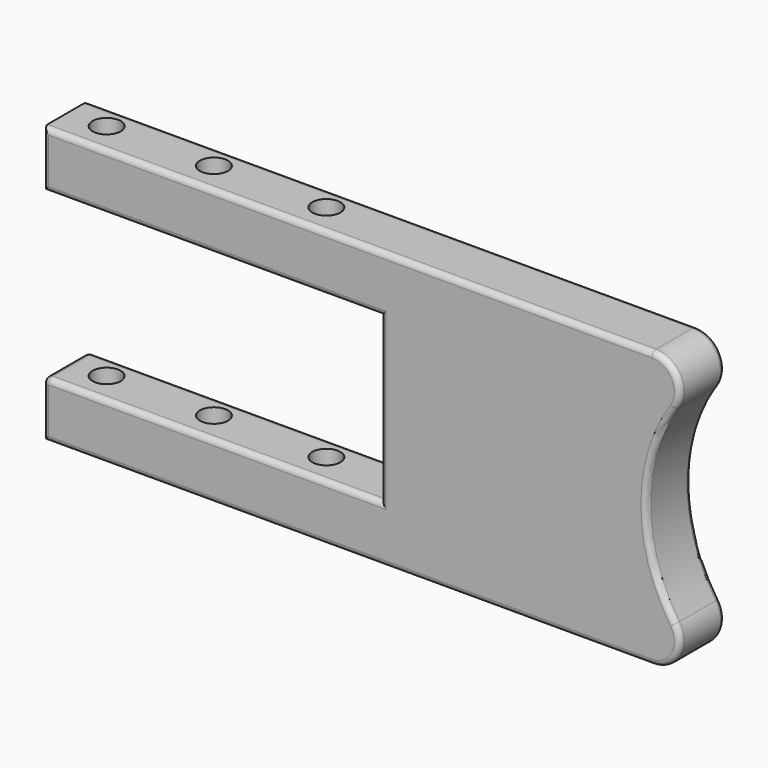
from build123d import *

# Parameters (mm, degrees)
F1_DEPTH     = 12.7
F2_R         = 6.35
F3_W         = 76.2
F3_H         = 36.9506594684
F4_DEPTH     = 12.701
F5_R         = 3.175
F6_DEPTH     = 62.3516594684
F7_T1_DEPTH  = 140.6081975657
F7_T3_DEPTH  = 79.3774143709
F7_T5_DEPTH  = 36.9506594684
F7_T7_DEPTH  = 74.9290343146
F7_T9_DEPTH  = 19.0548287418
F7_T11_DEPTH = 14.6064486855
F7_T13_DEPTH = 10.1580686292
F7_S17_W     = 1.3985022539
F7_S17_H     = 1.3985022539
F7_T18_DEPTH = 1.398502254
F7_S23_W     = 1.3985022539
F7_S23_H     = 1.3985022539
F7_T24_DEPTH = 1.398502254
F7_T40_ANGLE = 123.952133453
F7_T42_ANGLE = 67.904266906
F7_T44_ANGLE = 123.952133453
F7_T46_ANGLE = 123.952133453
F7_T48_ANGLE = 67.904266906
F7_T50_ANGLE = 123.952133453
F7_T55_DEPTH = 40.1280738393
F7_T59_DEPTH = 82.5548287418
F7_T66_DEPTH = 78.1064486855
F7_T70_DEPTH = 40.1280738393
F7_T77_DEPTH = 78.1064486855
F7_T81_DEPTH = 40.1280738393
F7_T88_DEPTH = 40.1280738393
F7_T92_DEPTH = 82.5548287418


# Not quite as in the source:
# - a fillet or chamfer that OpenCascade refuses, or shapes differently, is made with other operations: its cross-section is extruded or revolved along the edge and cut away or added


with BuildPart() as f1:
    # F0 (on Front) → F1 (new body)
    with BuildSketch(Plane.XZ):
        with BuildLine():
            Line((152.4, 62.3506594684), (0, 62.3506594684))
            Line((0, 62.3506594684), (0, 0))
            Line((0, 0), (152.4, 0))
            ThreePointArc((152.4, 0), (136.2022559561, 31.1753297342), (152.4, 62.3506594684))
        make_face()
    extrude(amount=F1_DEPTH)

    # F2
    f2_edges = [f1.edges().sort_by_distance(p)[0] for p in [
        (152.4, -6.35, 62.350659),
        (152.4, -6.35, 0),
    ]]
    fillet(f2_edges, radius=F2_R)

    # F3 (on face) → F4 (cut, through all)
    with BuildSketch(Plane.XZ.offset(12.7)):
        with Locations((38.1, 31.1753297342)):
            Rectangle(F3_W, F3_H)
    extrude(amount=-F4_DEPTH, mode=Mode.SUBTRACT)

    # F5 (on face) → F6 (cut, through all)
    with BuildSketch(Plane(origin=(0, 0, 0), x_dir=(1, 0, 0), z_dir=(0, 0, -1))):
        with Locations((58.1839601433, 5.4876524955)):
            Circle(F5_R)
        with Locations((32.7839601433, 5.4876524955)):
            Circle(F5_R)
        with Locations((8.5653553438, 5.4876524955)):
            Circle(F5_R)
    extrude(amount=-F6_DEPTH, mode=Mode.SUBTRACT)

    # F7: fillet of radius 1.27 on 19 edges, made by hand

    # F7_s2 → F7_t1 (cut)
    with BuildSketch(Plane.YZ.offset(-3.1774143709)):
        with BuildLine():
            ThreePointArc((-12.7004, 61.079693783), (-12.3280256121, 61.9786850805), (-11.4290343146, 62.3510594684))
            Line((-11.4290343146, 62.3510594684), (-11.4290343146, 62.4781960369))
            ThreePointArc((-11.4290343146, 62.4781960369), (-12.0645171573, 62.4777960369), (-12.7, 62.4777960369))
            Line((-12.7, 62.4777960369), (-12.8271365685, 62.3506594684))
            ThreePointArc((-12.8271365685, 62.3506594684), (-12.8271365685, 61.7151766257), (-12.8275365685, 61.079693783))
            Line((-12.8275365685, 61.079693783), (-12.7004, 61.079693783))
        make_face()
        with BuildLine():
            ThreePointArc((0.0004, 1.2709656854), (-0.3719743879, 0.3719743879), (-1.2709656854, -0.0004))
            Line((-1.2709656854, -0.0004), (-1.2709656854, -0.1275365685))
            ThreePointArc((-1.2709656854, -0.1275365685), (-0.6354828427, -0.1271365685), (0, -0.1271365685))
            Line((0, -0.1271365685), (0.1271365685, 0))
            ThreePointArc((0.1271365685, 0), (0.1271365685, 0.6354828427), (0.1275365685, 1.2709656854))
            Line((0.1275365685, 1.2709656854), (0.0004, 1.2709656854))
        make_face()
        with BuildLine():
            ThreePointArc((0.0004, 61.079693783), (-0.3719743879, 61.9786850805), (-1.2709656854, 62.3510594684))
            Line((-1.2709656854, 62.3510594684), (-1.2709656854, 62.4781960369))
            ThreePointArc((-1.2709656854, 62.4781960369), (-0.6354828427, 62.4777960369), (0, 62.4777960369))
            Line((0, 62.4777960369), (0.1271365685, 62.3506594684))
            ThreePointArc((0.1271365685, 62.3506594684), (0.1271365685, 61.7151766257), (0.1275365685, 61.079693783))
            Line((0.1275365685, 61.079693783), (0.0004, 61.079693783))
        make_face()
        with BuildLine():
            ThreePointArc((-12.7004, 1.2709656854), (-12.3280256121, 0.3719743879), (-11.4290343146, -0.0004))
            Line((-11.4290343146, -0.0004), (-11.4290343146, -0.1275365685))
            ThreePointArc((-11.4290343146, -0.1275365685), (-12.0645171573, -0.1271365685), (-12.7, -0.1271365685))
            Line((-12.7, -0.1271365685), (-12.8271365685, 0))
            ThreePointArc((-12.8271365685, 0), (-12.8271365685, 0.6354828427), (-12.8275365685, 1.2709656854))
            Line((-12.8275365685, 1.2709656854), (-12.7004, 1.2709656854))
        make_face()
    extrude(amount=F7_T1_DEPTH, mode=Mode.SUBTRACT)

    # F7_s4 → F7_t3 (cut)
    with BuildSketch(Plane.YZ.offset(-3.1774143709)):
        with BuildLine():
            ThreePointArc((-12.7004, 50.9216251538), (-12.3280256121, 50.0226338563), (-11.4290343146, 49.6502594684))
            Line((-11.4290343146, 49.6502594684), (-11.4290343146, 49.5231228998))
            ThreePointArc((-11.4290343146, 49.5231228998), (-12.0645171573, 49.5235228998), (-12.7, 49.5235228998))
            Line((-12.7, 49.5235228998), (-12.8271365685, 49.6506594684))
            ThreePointArc((-12.8271365685, 49.6506594684), (-12.8271365685, 50.2861423111), (-12.8275365685, 50.9216251538))
            Line((-12.8275365685, 50.9216251538), (-12.7004, 50.9216251538))
        make_face()
        with BuildLine():
            ThreePointArc((0.0004, 50.9216251538), (-0.3719743879, 50.0226338563), (-1.2709656854, 49.6502594684))
            Line((-1.2709656854, 49.6502594684), (-1.2709656854, 49.5231228998))
            ThreePointArc((-1.2709656854, 49.5231228998), (-0.6354828427, 49.5235228998), (0, 49.5235228998))
            Line((0, 49.5235228998), (0.1271365685, 49.6506594684))
            ThreePointArc((0.1271365685, 49.6506594684), (0.1271365685, 50.2861423111), (0.1275365685, 50.9216251538))
            Line((0.1275365685, 50.9216251538), (0.0004, 50.9216251538))
        make_face()
    extrude(amount=F7_T3_DEPTH, mode=Mode.SUBTRACT)

    # F7_s6 → F7_t5 (cut)
    with BuildSketch(Plane.XY.offset(12.7)):
        with BuildLine():
            ThreePointArc((77.4709656854, -12.7004), (76.5719743879, -12.3280256121), (76.1996, -11.4290343146))
            Line((76.1996, -11.4290343146), (76.0724634315, -11.4290343146))
            ThreePointArc((76.0724634315, -11.4290343146), (76.0728634315, -12.0645171573), (76.0728634315, -12.7))
            Line((76.0728634315, -12.7), (76.2, -12.8271365685))
            ThreePointArc((76.2, -12.8271365685), (76.8354828427, -12.8271365685), (77.4709656854, -12.8275365685))
            Line((77.4709656854, -12.8275365685), (77.4709656854, -12.7004))
        make_face()
        with BuildLine():
            ThreePointArc((77.4709656854, 0.0004), (76.5719743879, -0.3719743879), (76.1996, -1.2709656854))
            Line((76.1996, -1.2709656854), (76.0724634315, -1.2709656854))
            ThreePointArc((76.0724634315, -1.2709656854), (76.0728634315, -0.6354828427), (76.0728634315, 0))
            Line((76.0728634315, 0), (76.2, 0.1271365685))
            ThreePointArc((76.2, 0.1271365685), (76.8354828427, 0.1271365685), (77.4709656854, 0.1275365685))
            Line((77.4709656854, 0.1275365685), (77.4709656854, 0.0004))
        make_face()
    extrude(amount=F7_T5_DEPTH, mode=Mode.SUBTRACT)

    # F7_s8 → F7_t7 (cut)
    with BuildSketch(Plane.YZ.offset(1.2709656854)):
        with BuildLine():
            ThreePointArc((-12.7004, 11.4290343146), (-12.3280256121, 12.3280256121), (-11.4290343146, 12.7004))
            Line((-11.4290343146, 12.7004), (-11.4290343146, 12.8275365685))
            ThreePointArc((-11.4290343146, 12.8275365685), (-12.0645171573, 12.8271365685), (-12.7, 12.8271365685))
            Line((-12.7, 12.8271365685), (-12.8271365685, 12.7))
            ThreePointArc((-12.8271365685, 12.7), (-12.8271365685, 12.0645171573), (-12.8275365685, 11.4290343146))
            Line((-12.8275365685, 11.4290343146), (-12.7004, 11.4290343146))
        make_face()
        with BuildLine():
            ThreePointArc((0.0004, 11.4290343146), (-0.3719743879, 12.3280256121), (-1.2709656854, 12.7004))
            Line((-1.2709656854, 12.7004), (-1.2709656854, 12.8275365685))
            ThreePointArc((-1.2709656854, 12.8275365685), (-0.6354828427, 12.8271365685), (0, 12.8271365685))
            Line((0, 12.8271365685), (0.1271365685, 12.7))
            ThreePointArc((0.1271365685, 12.7), (0.1271365685, 12.0645171573), (0.1275365685, 11.4290343146))
            Line((0.1275365685, 11.4290343146), (0.0004, 11.4290343146))
        make_face()
    extrude(amount=F7_T7_DEPTH, mode=Mode.SUBTRACT)

    # F7_s10 → F7_t9 (cut)
    with BuildSketch(Plane.XY.offset(46.4732450975)):
        with BuildLine():
            ThreePointArc((1.2709656854, -12.7004), (0.3719743879, -12.3280256121), (-0.0004, -11.4290343146))
            Line((-0.0004, -11.4290343146), (-0.1275365685, -11.4290343146))
            ThreePointArc((-0.1275365685, -11.4290343146), (-0.1271365685, -12.0645171573), (-0.1271365685, -12.7))
            Line((-0.1271365685, -12.7), (0, -12.8271365685))
            ThreePointArc((0, -12.8271365685), (0.6354828427, -12.8271365685), (1.2709656854, -12.8275365685))
            Line((1.2709656854, -12.8275365685), (1.2709656854, -12.7004))
        make_face()
        with BuildLine():
            ThreePointArc((1.2709656854, 0.0004), (0.3719743879, -0.3719743879), (-0.0004, -1.2709656854))
            Line((-0.0004, -1.2709656854), (-0.1275365685, -1.2709656854))
            ThreePointArc((-0.1275365685, -1.2709656854), (-0.1271365685, -0.6354828427), (-0.1271365685, 0))
            Line((-0.1271365685, 0), (0, 0.1271365685))
            ThreePointArc((0, 0.1271365685), (0.6354828427, 0.1271365685), (1.2709656854, 0.1275365685))
            Line((1.2709656854, 0.1275365685), (1.2709656854, 0.0004))
        make_face()
    extrude(amount=F7_T9_DEPTH, mode=Mode.SUBTRACT)

    # F7_s12 → F7_t11 (cut)
    with BuildSketch(Plane.XY.offset(-3.1774143709)):
        with BuildLine():
            ThreePointArc((1.2709656854, -12.7004), (0.3719743879, -12.3280256121), (-0.0004, -11.4290343146))
            Line((-0.0004, -11.4290343146), (-0.1275365685, -11.4290343146))
            ThreePointArc((-0.1275365685, -11.4290343146), (-0.1271365685, -12.0645171573), (-0.1271365685, -12.7))
            Line((-0.1271365685, -12.7), (0, -12.8271365685))
            ThreePointArc((0, -12.8271365685), (0.6354828427, -12.8271365685), (1.2709656854, -12.8275365685))
            Line((1.2709656854, -12.8275365685), (1.2709656854, -12.7004))
        make_face()
        with BuildLine():
            ThreePointArc((1.2709656854, 0.0004), (0.3719743879, -0.3719743879), (-0.0004, -1.2709656854))
            Line((-0.0004, -1.2709656854), (-0.1275365685, -1.2709656854))
            ThreePointArc((-0.1275365685, -1.2709656854), (-0.1271365685, -0.6354828427), (-0.1271365685, 0))
            Line((-0.1271365685, 0), (0, 0.1271365685))
            ThreePointArc((0, 0.1271365685), (0.6354828427, 0.1271365685), (1.2709656854, 0.1275365685))
            Line((1.2709656854, 0.1275365685), (1.2709656854, 0.0004))
        make_face()
    extrude(amount=F7_T11_DEPTH, mode=Mode.SUBTRACT)

    # F7_s14 → F7_t13 (cut)
    with BuildSketch(Plane.XZ.offset(1.2709656854)):
        with BuildLine():
            ThreePointArc((-0.0004, 11.4290343146), (0.3719743879, 12.3280256121), (1.2709656854, 12.7004))
            Line((1.2709656854, 12.7004), (1.2709656854, 12.8275365685))
            ThreePointArc((1.2709656854, 12.8275365685), (0.6354828427, 12.8271365685), (0, 12.8271365685))
            Line((0, 12.8271365685), (-0.1271365685, 12.7))
            ThreePointArc((-0.1271365685, 12.7), (-0.1271365685, 12.0645171573), (-0.1275365685, 11.4290343146))
            Line((-0.1275365685, 11.4290343146), (-0.0004, 11.4290343146))
        make_face()
    extrude(amount=F7_T13_DEPTH, mode=Mode.SUBTRACT)


with BuildPart() as f7_tool16:
    # F7_s17 → F7_t18 (new body)
    with BuildSketch(Plane.XZ.offset(11.4290343146)):
        with Locations((0.5717145584, 12.1282854416)):
            Rectangle(F7_S17_W, F7_S17_H)
    extrude(amount=F7_T18_DEPTH)

    # F7_s19 → F7_t20 (revolve, cut)
    with BuildSketch(Plane(origin=(1.2709656854, -11.4290343146, 11.4290343146), x_dir=(0.7071067812, 0, -0.7071067812), z_dir=(-0.7071067812, 0, -0.7071067812))):
        with BuildLine():
            ThreePointArc((0, -1.2713656854), (1.2713656854, 0), (0, 1.2713656854))
            Line((0, 1.2713656854), (0, -1.2713656854))
        make_face()
    revolve(axis=Axis((1.2709656854, -11.4290343146, 11.4290343146), (0, -1, 0)), mode=Mode.SUBTRACT)


with BuildPart() as f1_1:
    add(f1.part)

    # F7_t15: cut F7_tool16
    add(f7_tool16.part, mode=Mode.SUBTRACT)


with BuildPart() as f7_tool22:
    # F7_s23 → F7_t24 (new body)
    with BuildSketch(Plane.XZ.offset(1.2709656854)):
        with Locations((0.5717145584, 12.1282854416)):
            Rectangle(F7_S23_W, F7_S23_H)
    extrude(amount=-F7_T24_DEPTH)

    # F7_s25 → F7_t26 (revolve, cut)
    with BuildSketch(Plane(origin=(1.2709656854, -1.2709656854, 11.4290343146), x_dir=(0.7071067812, 0, -0.7071067812), z_dir=(0.7071067812, 0, 0.7071067812))):
        with BuildLine():
            ThreePointArc((0, -1.2713656854), (1.2713656854, 0), (0, 1.2713656854))
            Line((0, 1.2713656854), (0, -1.2713656854))
        make_face()
    revolve(axis=Axis((1.2709656854, -1.2709656854, 11.4290343146), (0, 1, 0)), mode=Mode.SUBTRACT)


with BuildPart() as f1_2:
    add(f1_1.part)

    # F7_t21: cut F7_tool22
    add(f7_tool22.part, mode=Mode.SUBTRACT)

    # F7_s27 → F7_t28 (revolve, cut)
    with BuildSketch(Plane.XZ.offset(5.4876524955)):
        with BuildLine():
            ThreePointArc((62.6299258287, -0.0004), (61.7309345312, 0.3719743879), (61.3585601433, 1.2709656854))
            Line((61.3585601433, 1.2709656854), (61.2314235747, 1.2709656854))
            ThreePointArc((61.2314235747, 1.2709656854), (61.2318235747, 0.6354828427), (61.2318235747, 0))
            Line((61.2318235747, 0), (61.3589601433, -0.1271365685))
            ThreePointArc((61.3589601433, -0.1271365685), (61.994442986, -0.1271365685), (62.6299258287, -0.1275365685))
            Line((62.6299258287, -0.1275365685), (62.6299258287, -0.0004))
        make_face()
    revolve(axis=Axis((58.1839601433, -5.4876524955, 0), (0, 0, -1)), mode=Mode.SUBTRACT)

    # F7_s29 → F7_t30 (revolve, cut)
    with BuildSketch(Plane.XZ.offset(5.4876524955)):
        with BuildLine():
            ThreePointArc((37.2299258287, -0.0004), (36.3309345312, 0.3719743879), (35.9585601433, 1.2709656854))
            Line((35.9585601433, 1.2709656854), (35.8314235747, 1.2709656854))
            ThreePointArc((35.8314235747, 1.2709656854), (35.8318235747, 0.6354828427), (35.8318235747, 0))
            Line((35.8318235747, 0), (35.9589601433, -0.1271365685))
            ThreePointArc((35.9589601433, -0.1271365685), (36.594442986, -0.1271365685), (37.2299258287, -0.1275365685))
            Line((37.2299258287, -0.1275365685), (37.2299258287, -0.0004))
        make_face()
    revolve(axis=Axis((32.7839601433, -5.4876524955, 0), (0, 0, -1)), mode=Mode.SUBTRACT)

    # F7_s31 → F7_t32 (revolve, cut)
    with BuildSketch(Plane.XZ.offset(5.4876524955)):
        with BuildLine():
            ThreePointArc((13.0113210292, -0.0004), (12.1123297316, 0.3719743879), (11.7399553438, 1.2709656854))
            Line((11.7399553438, 1.2709656854), (11.6128187752, 1.2709656854))
            ThreePointArc((11.6128187752, 1.2709656854), (11.6132187752, 0.6354828427), (11.6132187752, 0))
            Line((11.6132187752, 0), (11.7403553438, -0.1271365685))
            ThreePointArc((11.7403553438, -0.1271365685), (12.3758381865, -0.1271365685), (13.0113210292, -0.1275365685))
            Line((13.0113210292, -0.1275365685), (13.0113210292, -0.0004))
        make_face()
    revolve(axis=Axis((8.5653553438, -5.4876524955, 0), (0, 0, -1)), mode=Mode.SUBTRACT)

    # F7_s33 → F7_t34 (revolve, cut)
    with BuildSketch(Plane.XZ.offset(5.4876524955)):
        with BuildLine():
            ThreePointArc((62.6299258287, 49.6502594684), (61.7309345312, 50.0226338563), (61.3585601433, 50.9216251538))
            Line((61.3585601433, 50.9216251538), (61.2314235747, 50.9216251538))
            ThreePointArc((61.2314235747, 50.9216251538), (61.2318235747, 50.2861423111), (61.2318235747, 49.6506594684))
            Line((61.2318235747, 49.6506594684), (61.3589601433, 49.5235228998))
            ThreePointArc((61.3589601433, 49.5235228998), (61.994442986, 49.5235228998), (62.6299258287, 49.5231228998))
            Line((62.6299258287, 49.5231228998), (62.6299258287, 49.6502594684))
        make_face()
    revolve(axis=Axis((58.1839601433, -5.4876524955, 49.6506594684), (0, 0, -1)), mode=Mode.SUBTRACT)

    # F7_s35 → F7_t36 (revolve, cut)
    with BuildSketch(Plane.XZ.offset(5.4876524955)):
        with BuildLine():
            ThreePointArc((37.2299258287, 49.6502594684), (36.3309345312, 50.0226338563), (35.9585601433, 50.9216251538))
            Line((35.9585601433, 50.9216251538), (35.8314235747, 50.9216251538))
            ThreePointArc((35.8314235747, 50.9216251538), (35.8318235747, 50.2861423111), (35.8318235747, 49.6506594684))
            Line((35.8318235747, 49.6506594684), (35.9589601433, 49.5235228998))
            ThreePointArc((35.9589601433, 49.5235228998), (36.594442986, 49.5235228998), (37.2299258287, 49.5231228998))
            Line((37.2299258287, 49.5231228998), (37.2299258287, 49.6502594684))
        make_face()
    revolve(axis=Axis((32.7839601433, -5.4876524955, 49.6506594684), (0, 0, -1)), mode=Mode.SUBTRACT)

    # F7_s37 → F7_t38 (revolve, cut)
    with BuildSketch(Plane.XZ.offset(5.4876524955)):
        with BuildLine():
            ThreePointArc((13.0113210292, 49.6502594684), (12.1123297316, 50.0226338563), (11.7399553438, 50.9216251538))
            Line((11.7399553438, 50.9216251538), (11.6128187752, 50.9216251538))
            ThreePointArc((11.6128187752, 50.9216251538), (11.6132187752, 50.2861423111), (11.6132187752, 49.6506594684))
            Line((11.6132187752, 49.6506594684), (11.7403553438, 49.5235228998))
            ThreePointArc((11.7403553438, 49.5235228998), (12.3758381865, 49.5235228998), (13.0113210292, 49.5231228998))
            Line((13.0113210292, 49.5231228998), (13.0113210292, 49.6502594684))
        make_face()
    revolve(axis=Axis((8.5653553438, -5.4876524955, 49.6506594684), (0, 0, -1)), mode=Mode.SUBTRACT)

    # F7_s39 → F7_t40 (revolve, cut)
    with BuildSketch(Plane(origin=(39.9259181111, 0, -59.2994098312), x_dir=(0, 1, 0), z_dir=(-0.5585001065, 0, 0.8295044491))):
        with BuildLine():
            ThreePointArc((0.0004, -122.6249560906), (-0.3719743879, -123.5239473881), (-1.2709656854, -123.896321776))
            Line((-1.2709656854, -123.896321776), (-1.2709656854, -124.0234583445))
            ThreePointArc((-1.2709656854, -124.0234583445), (-0.6354828427, -124.0230583445), (0, -124.0230583445))
            Line((0, -124.0230583445), (0.1271365685, -123.895921776))
            ThreePointArc((0.1271365685, -123.895921776), (0.1271365685, -123.2604389333), (0.1275365685, -122.6249560906))
            Line((0.1275365685, -122.6249560906), (0.0004, -122.6249560906))
        make_face()
    revolve(axis=Axis((137.4307831947, 0, 6.35), (0, 1, 0)), revolution_arc=F7_T40_ANGLE, mode=Mode.SUBTRACT)

    # F7_s41 → F7_t42 (revolve, cut)
    with BuildSketch(Plane(origin=(39.9259181111, 0, -59.2994098312), x_dir=(0, 1, 0), z_dir=(0.5585001065, 0, -0.8295044491))):
        with BuildLine():
            ThreePointArc((-1.2709656854, 123.896321776), (-0.3719743879, 123.5239473881), (0.0004, 122.6249560906))
            Line((0.0004, 122.6249560906), (0.1275365685, 122.6249560906))
            ThreePointArc((0.1275365685, 122.6249560906), (0.1271365685, 123.2604389333), (0.1271365685, 123.895921776))
            Line((0.1271365685, 123.895921776), (0, 124.0230583445))
            ThreePointArc((0, 124.0230583445), (-0.6354828427, 124.0230583445), (-1.2709656854, 124.0234583445))
            Line((-1.2709656854, 124.0234583445), (-1.2709656854, 123.896321776))
        make_face()
    revolve(axis=Axis((174.3022559561, 0, 31.1753297342), (0, 1, 0)), revolution_arc=F7_T42_ANGLE, mode=Mode.SUBTRACT)

    # F7_s43 → F7_t44 (revolve, cut)
    with BuildSketch(Plane(origin=(68.8116270772, 0, 102.2015038916), x_dir=(0, 1, 0), z_dir=(-0.5585001065, 0, -0.8295044491))):
        with BuildLine():
            ThreePointArc((0.0004, 87.8021061368), (-0.3719743879, 88.7010974343), (-1.2709656854, 89.0734718222))
            Line((-1.2709656854, 89.0734718222), (-1.2709656854, 89.2006083907))
            ThreePointArc((-1.2709656854, 89.2006083907), (-0.6354828427, 89.2002083907), (0, 89.2002083907))
            Line((0, 89.2002083907), (0.1271365685, 89.0730718222))
            ThreePointArc((0.1271365685, 89.0730718222), (0.1271365685, 88.4375889795), (0.1275365685, 87.8021061368))
            Line((0.1275365685, 87.8021061368), (0.0004, 87.8021061368))
        make_face()
    revolve(axis=Axis((137.4307831947, 0, 56.0006594684), (0, -1, 0)), revolution_arc=F7_T44_ANGLE, mode=Mode.SUBTRACT)

    # F7_s45 → F7_t46 (revolve, cut)
    with BuildSketch(Plane(origin=(68.8116270772, 0, 102.2015038916), x_dir=(0, 1, 0), z_dir=(-0.5585001065, 0, -0.8295044491))):
        with BuildLine():
            ThreePointArc((-11.4290343146, 89.0734718222), (-12.3280256121, 88.7010974343), (-12.7004, 87.8021061368))
            Line((-12.7004, 87.8021061368), (-12.8275365685, 87.8021061368))
            ThreePointArc((-12.8275365685, 87.8021061368), (-12.8271365685, 88.4375889795), (-12.8271365685, 89.0730718222))
            Line((-12.8271365685, 89.0730718222), (-12.7, 89.2002083907))
            ThreePointArc((-12.7, 89.2002083907), (-12.0645171573, 89.2002083907), (-11.4290343146, 89.2006083907))
            Line((-11.4290343146, 89.2006083907), (-11.4290343146, 89.0734718222))
        make_face()
    revolve(axis=Axis((137.4307831947, -12.7, 56.0006594684), (0, -1, 0)), revolution_arc=F7_T46_ANGLE, mode=Mode.SUBTRACT)

    # F7_s47 → F7_t48 (revolve, cut)
    with BuildSketch(Plane(origin=(39.9259181111, 0, -59.2994098312), x_dir=(0, 1, 0), z_dir=(0.5585001065, 0, -0.8295044491))):
        with BuildLine():
            ThreePointArc((-11.4290343146, 123.896321776), (-12.3280256121, 123.5239473881), (-12.7004, 122.6249560906))
            Line((-12.7004, 122.6249560906), (-12.8275365685, 122.6249560906))
            ThreePointArc((-12.8275365685, 122.6249560906), (-12.8271365685, 123.2604389333), (-12.8271365685, 123.895921776))
            Line((-12.8271365685, 123.895921776), (-12.7, 124.0230583445))
            ThreePointArc((-12.7, 124.0230583445), (-12.0645171573, 124.0230583445), (-11.4290343146, 124.0234583445))
            Line((-11.4290343146, 124.0234583445), (-11.4290343146, 123.896321776))
        make_face()
    revolve(axis=Axis((174.3022559561, -12.7, 31.1753297342), (0, 1, 0)), revolution_arc=F7_T48_ANGLE, mode=Mode.SUBTRACT)

    # F7_s49 → F7_t50 (revolve, cut)
    with BuildSketch(Plane(origin=(39.9259181111, 0, -59.2994098312), x_dir=(0, 1, 0), z_dir=(-0.5585001065, 0, 0.8295044491))):
        with BuildLine():
            ThreePointArc((-11.4290343146, -123.896321776), (-12.3280256121, -123.5239473881), (-12.7004, -122.6249560906))
            Line((-12.7004, -122.6249560906), (-12.8275365685, -122.6249560906))
            ThreePointArc((-12.8275365685, -122.6249560906), (-12.8271365685, -123.2604389333), (-12.8271365685, -123.895921776))
            Line((-12.8271365685, -123.895921776), (-12.7, -124.0230583445))
            ThreePointArc((-12.7, -124.0230583445), (-12.0645171573, -124.0230583445), (-11.4290343146, -124.0234583445))
            Line((-11.4290343146, -124.0234583445), (-11.4290343146, -123.896321776))
        make_face()
    revolve(axis=Axis((137.4307831947, -12.7, 6.35), (0, 1, 0)), revolution_arc=F7_T50_ANGLE, mode=Mode.SUBTRACT)


with BuildPart() as f7_tool53:
    # F7_s54 → F7_t55 (new body)
    with BuildSketch(Plane.XY.offset(12.7)):
        with BuildLine():
            ThreePointArc((77.4709656854, -12.7004), (76.5719743879, -12.3280256121), (76.1996, -11.4290343146))
            Line((76.1996, -11.4290343146), (76.0724634315, -11.4290343146))
            ThreePointArc((76.0724634315, -11.4290343146), (76.0728634315, -12.0645171573), (76.0728634315, -12.7))
            Line((76.0728634315, -12.7), (76.2, -12.8271365685))
            ThreePointArc((76.2, -12.8271365685), (76.8354828427, -12.8271365685), (77.4709656854, -12.8275365685))
            Line((77.4709656854, -12.8275365685), (77.4709656854, -12.7004))
        make_face()
    extrude(amount=F7_T55_DEPTH)

    split(bisect_by=Plane.XY.offset(49.6506594684), keep=Keep.TOP)


with BuildPart() as f7_tool57:
    # F7_s58 → F7_t59 (new body)
    with BuildSketch(Plane.YZ.offset(79.3774143709)):
        with BuildLine():
            ThreePointArc((-12.7004, 50.9216251538), (-12.3280256121, 50.0226338563), (-11.4290343146, 49.6502594684))
            Line((-11.4290343146, 49.6502594684), (-11.4290343146, 49.5231228998))
            ThreePointArc((-11.4290343146, 49.5231228998), (-12.0645171573, 49.5235228998), (-12.7, 49.5235228998))
            Line((-12.7, 49.5235228998), (-12.8271365685, 49.6506594684))
            ThreePointArc((-12.8271365685, 49.6506594684), (-12.8271365685, 50.2861423111), (-12.8275365685, 50.9216251538))
            Line((-12.8275365685, 50.9216251538), (-12.7004, 50.9216251538))
        make_face()
    extrude(amount=-F7_T59_DEPTH)

    split(bisect_by=Plane.YZ.offset(76.2), keep=Keep.TOP)


with BuildPart() as f7_tool53_1:
    add(f7_tool53.part)

    # F7_t61: intersect F7_tool57
    add(f7_tool57.part, mode=Mode.INTERSECT)


with BuildPart() as f1_3:
    add(f1_2.part)

    # F7_t51: cut F7_tool53
    add(f7_tool53_1.part, mode=Mode.SUBTRACT)


with BuildPart() as f7_tool64:
    # F7_s65 → F7_t66 (new body)
    with BuildSketch(Plane.YZ.offset(1.2709656854)):
        with BuildLine():
            ThreePointArc((-12.7004, 11.4290343146), (-12.3280256121, 12.3280256121), (-11.4290343146, 12.7004))
            Line((-11.4290343146, 12.7004), (-11.4290343146, 12.8275365685))
            ThreePointArc((-11.4290343146, 12.8275365685), (-12.0645171573, 12.8271365685), (-12.7, 12.8271365685))
            Line((-12.7, 12.8271365685), (-12.8271365685, 12.7))
            ThreePointArc((-12.8271365685, 12.7), (-12.8271365685, 12.0645171573), (-12.8275365685, 11.4290343146))
            Line((-12.8275365685, 11.4290343146), (-12.7004, 11.4290343146))
        make_face()
    extrude(amount=F7_T66_DEPTH)

    split(bisect_by=Plane.YZ.offset(76.2), keep=Keep.TOP)


with BuildPart() as f7_tool68:
    # F7_s69 → F7_t70 (new body)
    with BuildSketch(Plane.XY.offset(9.5225856291)):
        with BuildLine():
            ThreePointArc((77.4709656854, -12.7004), (76.5719743879, -12.3280256121), (76.1996, -11.4290343146))
            Line((76.1996, -11.4290343146), (76.0724634315, -11.4290343146))
            ThreePointArc((76.0724634315, -11.4290343146), (76.0728634315, -12.0645171573), (76.0728634315, -12.7))
            Line((76.0728634315, -12.7), (76.2, -12.8271365685))
            ThreePointArc((76.2, -12.8271365685), (76.8354828427, -12.8271365685), (77.4709656854, -12.8275365685))
            Line((77.4709656854, -12.8275365685), (77.4709656854, -12.7004))
        make_face()
    extrude(amount=F7_T70_DEPTH)

    split(bisect_by=Plane.XY.offset(12.7), keep=Keep.BOTTOM)


with BuildPart() as f7_tool64_1:
    add(f7_tool64.part)

    # F7_t72: intersect F7_tool68
    add(f7_tool68.part, mode=Mode.INTERSECT)


with BuildPart() as f1_4:
    add(f1_3.part)

    # F7_t62: cut F7_tool64
    add(f7_tool64_1.part, mode=Mode.SUBTRACT)


with BuildPart() as f7_tool75:
    # F7_s76 → F7_t77 (new body)
    with BuildSketch(Plane.YZ.offset(1.2709656854)):
        with BuildLine():
            ThreePointArc((0.0004, 11.4290343146), (-0.3719743879, 12.3280256121), (-1.2709656854, 12.7004))
            Line((-1.2709656854, 12.7004), (-1.2709656854, 12.8275365685))
            ThreePointArc((-1.2709656854, 12.8275365685), (-0.6354828427, 12.8271365685), (0, 12.8271365685))
            Line((0, 12.8271365685), (0.1271365685, 12.7))
            ThreePointArc((0.1271365685, 12.7), (0.1271365685, 12.0645171573), (0.1275365685, 11.4290343146))
            Line((0.1275365685, 11.4290343146), (0.0004, 11.4290343146))
        make_face()
    extrude(amount=F7_T77_DEPTH)

    split(bisect_by=Plane.YZ.offset(76.2), keep=Keep.TOP)


with BuildPart() as f7_tool79:
    # F7_s80 → F7_t81 (new body)
    with BuildSketch(Plane.XY.offset(9.5225856291)):
        with BuildLine():
            ThreePointArc((77.4709656854, 0.0004), (76.5719743879, -0.3719743879), (76.1996, -1.2709656854))
            Line((76.1996, -1.2709656854), (76.0724634315, -1.2709656854))
            ThreePointArc((76.0724634315, -1.2709656854), (76.0728634315, -0.6354828427), (76.0728634315, 0))
            Line((76.0728634315, 0), (76.2, 0.1271365685))
            ThreePointArc((76.2, 0.1271365685), (76.8354828427, 0.1271365685), (77.4709656854, 0.1275365685))
            Line((77.4709656854, 0.1275365685), (77.4709656854, 0.0004))
        make_face()
    extrude(amount=F7_T81_DEPTH)

    split(bisect_by=Plane.XY.offset(12.7), keep=Keep.BOTTOM)


with BuildPart() as f7_tool75_1:
    add(f7_tool75.part)

    # F7_t83: intersect F7_tool79
    add(f7_tool79.part, mode=Mode.INTERSECT)


with BuildPart() as f1_5:
    add(f1_4.part)

    # F7_t73: cut F7_tool75
    add(f7_tool75_1.part, mode=Mode.SUBTRACT)


with BuildPart() as f7_tool86:
    # F7_s87 → F7_t88 (new body)
    with BuildSketch(Plane.XY.offset(12.7)):
        with BuildLine():
            ThreePointArc((77.4709656854, 0.0004), (76.5719743879, -0.3719743879), (76.1996, -1.2709656854))
            Line((76.1996, -1.2709656854), (76.0724634315, -1.2709656854))
            ThreePointArc((76.0724634315, -1.2709656854), (76.0728634315, -0.6354828427), (76.0728634315, 0))
            Line((76.0728634315, 0), (76.2, 0.1271365685))
            ThreePointArc((76.2, 0.1271365685), (76.8354828427, 0.1271365685), (77.4709656854, 0.1275365685))
            Line((77.4709656854, 0.1275365685), (77.4709656854, 0.0004))
        make_face()
    extrude(amount=F7_T88_DEPTH)

    split(bisect_by=Plane.XY.offset(49.6506594684), keep=Keep.TOP)


with BuildPart() as f7_tool90:
    # F7_s91 → F7_t92 (new body)
    with BuildSketch(Plane.YZ.offset(79.3774143709)):
        with BuildLine():
            ThreePointArc((0.0004, 50.9216251538), (-0.3719743879, 50.0226338563), (-1.2709656854, 49.6502594684))
            Line((-1.2709656854, 49.6502594684), (-1.2709656854, 49.5231228998))
            ThreePointArc((-1.2709656854, 49.5231228998), (-0.6354828427, 49.5235228998), (0, 49.5235228998))
            Line((0, 49.5235228998), (0.1271365685, 49.6506594684))
            ThreePointArc((0.1271365685, 49.6506594684), (0.1271365685, 50.2861423111), (0.1275365685, 50.9216251538))
            Line((0.1275365685, 50.9216251538), (0.0004, 50.9216251538))
        make_face()
    extrude(amount=-F7_T92_DEPTH)

    split(bisect_by=Plane.YZ.offset(76.2), keep=Keep.TOP)


with BuildPart() as f7_tool86_1:
    add(f7_tool86.part)

    # F7_t94: intersect F7_tool90
    add(f7_tool90.part, mode=Mode.INTERSECT)


with BuildPart() as f1_6:
    add(f1_5.part)

    # F7_t84: cut F7_tool86
    add(f7_tool86_1.part, mode=Mode.SUBTRACT)


solid = f1_6.part
